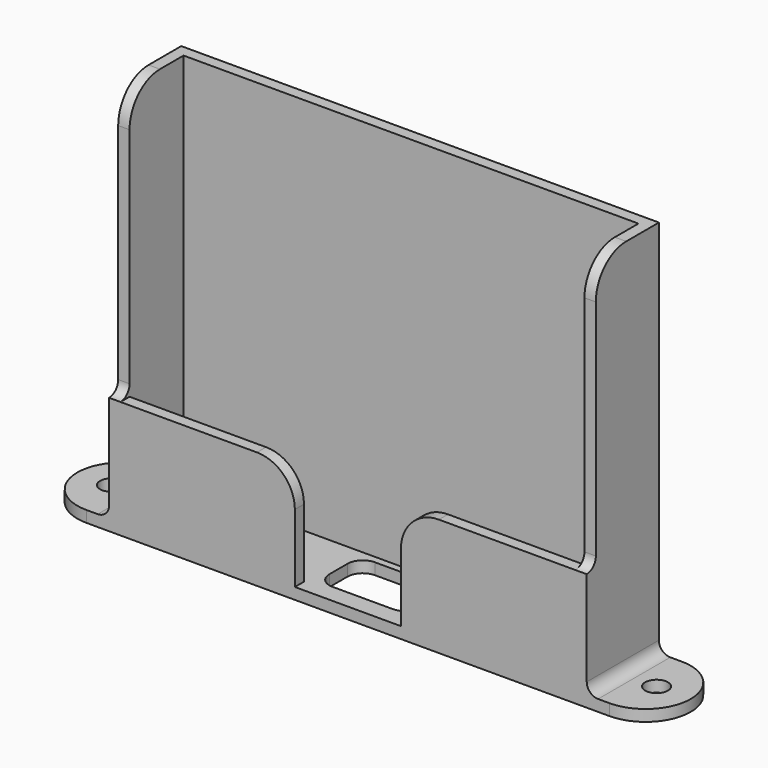
from build123d import *

# Parameters (mm, degrees)
F1_W        = 14
F1_H        = 1.5
F1_R        = 1.5
F2_DEPTH    = 1.5
F3_DEPTH    = 14
F4_DEPTH    = 50
F5_R        = 5
F6_T1_DEPTH = 1.5
F6_T3_DEPTH = 11.9
F6_T5_DEPTH = 1.5


# Not quite as in the source:
# - a fillet or chamfer that OpenCascade refuses, or shapes differently, is made with other operations: its cross-section is extruded or revolved along the edge and cut away or added
# - a feature names something its author has since deleted; it is built from what else it names


with BuildPart() as f2:
    # F1 (on Top) → F2 (new body)
    with BuildSketch(Plane.XY):
        Polygon((-61.5, -10.4), (-61.5, -1.5), (-1.5, -1.5), (-1.5, -10.4), (0, -10.4), (0, 0), (-63, 0), (-63, -10.4), align=None)
        Polygon((-38.5, -10.4), (-61.5, -10.4), (-63, -10.4), (-63, -11.9), (-38.5, -11.9), align=None)
        with Locations((-31.5, -11.15)):
            Rectangle(F1_W, F1_H)
        Polygon((0, -10.4), (-1.5, -10.4), (-24.5, -10.4), (-24.5, -11.9), (0, -11.9), align=None)
        Polygon((-1.5, -1.5), (-61.5, -1.5), (-61.5, -10.4), (-38.5, -10.4), (-24.5, -10.4), (-1.5, -10.4), align=None)
        with BuildLine():
            ThreePointArc((-37.5, -4.45), (-36.9142135624, -3.0357864376), (-35.5, -2.45))
            Line((-35.5, -2.45), (-27.5, -2.45))
            ThreePointArc((-27.5, -2.45), (-26.0857864376, -3.0357864376), (-25.5, -4.45))
            Line((-25.5, -4.45), (-25.5, -7.45))
            ThreePointArc((-25.5, -7.45), (-26.0857864376, -8.8642135624), (-27.5, -9.45))
            Line((-27.5, -9.45), (-35.5, -9.45))
            ThreePointArc((-35.5, -9.45), (-36.9142135624, -8.8642135624), (-37.5, -7.45))
            Line((-37.5, -7.45), (-37.5, -4.45))
        make_face(mode=Mode.SUBTRACT)
        with BuildLine():
            Line((-63, -11.9), (-63, -10.4))
            Line((-63, -10.4), (-63, 0))
            Line((-63, 0), (-66, 0))
            ThreePointArc((-66, 0), (-71.95, -5.95), (-66, -11.9))
            Line((-66, -11.9), (-63, -11.9))
        make_face()
        with Locations((-67.45, -5.95)):
            Circle(F1_R, mode=Mode.SUBTRACT)
        with BuildLine():
            Line((0, 0), (0, -10.4))
            Line((0, -10.4), (0, -11.9))
            Line((0, -11.9), (3, -11.9))
            ThreePointArc((3, -11.9), (8.95, -5.95), (3, 0))
            Line((3, 0), (0, 0))
        make_face()
        with Locations((4.45, -5.95)):
            Circle(F1_R, mode=Mode.SUBTRACT)
    extrude(amount=-F2_DEPTH)

    # F1 (on Top) → F3 (join)
    with BuildSketch(Plane.XY):
        Polygon((0, -10.4), (-1.5, -10.4), (-24.5, -10.4), (-24.5, -11.9), (0, -11.9), align=None)
        Polygon((-38.5, -10.4), (-61.5, -10.4), (-63, -10.4), (-63, -11.9), (-38.5, -11.9), align=None)
    extrude(amount=F3_DEPTH)

    # F1 (on Top) → F4 (join)
    with BuildSketch(Plane.XY):
        Polygon((-61.5, -10.4), (-61.5, -1.5), (-1.5, -1.5), (-1.5, -10.4), (0, -10.4), (0, 0), (-63, 0), (-63, -10.4), align=None)
    extrude(amount=F4_DEPTH)

    # F5
    f5_edges = [f2.edges().sort_by_distance(p)[0] for p in [
        (-62.25, -10.4, 50),
        (-0.75, -10.4, 50),
        (-24.5, -11.15, 14),
        (-38.5, -11.15, 14),
    ]]
    fillet(f5_edges, radius=F5_R)

    # F6: fillet of radius 1.5 on 4 edges, made by hand

    # F6_s2 → F6_t1 (join)
    with BuildSketch(Plane.YZ.offset(-63)):
        with BuildLine():
            ThreePointArc((-10.4, 15.5), (-10.8393398282, 14.4393398282), (-11.9, 14))
            Line((-11.9, 14), (-10.4, 14))
            Line((-10.4, 14), (-10.4, 15.5))
        make_face()
    extrude(amount=F6_T1_DEPTH)

    # F6_s4 → F6_t3 (join)
    with BuildSketch(Plane.XZ):
        with BuildLine():
            ThreePointArc((-63, 1.5), (-63.4393398282, 0.4393398282), (-64.5, 0))
            Line((-64.5, 0), (-63, 0))
            Line((-63, 0), (-63, 1.5))
        make_face()
        with BuildLine():
            ThreePointArc((0, 1.5), (0.4393398282, 0.4393398282), (1.5, 0))
            Line((1.5, 0), (0, 0))
            Line((0, 0), (0, 1.5))
        make_face()
    extrude(amount=F6_T3_DEPTH)

    # F6_s6 → F6_t5 (join)
    with BuildSketch(Plane.YZ.offset(-1.5)):
        with BuildLine():
            ThreePointArc((-10.4, 15.5), (-10.8393398282, 14.4393398282), (-11.9, 14))
            Line((-11.9, 14), (-10.4, 14))
            Line((-10.4, 14), (-10.4, 15.5))
        make_face()
    extrude(amount=F6_T5_DEPTH)


solid = f2.part
